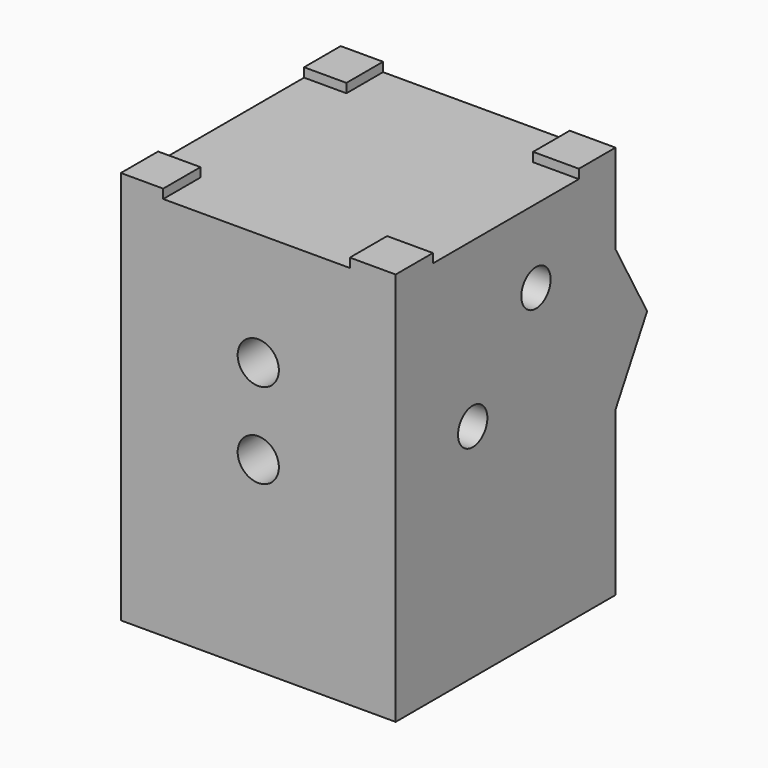
from build123d import *

# Parameters (mm, degrees)
F0_W      = 30
F0_H      = 30
F1_DEPTH  = 42
F5_R      = 2
F6_DEPTH  = 50
F8_R      = 2.25
F9_DEPTH  = 8
F10_R     = 2.25
F11_DEPTH = 16
F12_W     = 5
F12_H     = 5
F12_H_2   = 5.0838639587
F12_W_2   = 4.6232988685
F13_DEPTH = 1
F16_DEPTH = 20
F21_R     = 6.9
F2_R      = 6.75
F23_R     = 2.25
F24_DEPTH = 8.5855845434
F26_DEPTH = 30


with BuildPart() as f1:
    # F0 (on Top) → F1 (new body)
    with BuildSketch(Plane.XY):
        Rectangle(F0_W, F0_H)
    extrude(amount=F1_DEPTH)

    # F5 (on offset) → F6 (cut)
    with BuildSketch(Plane.YZ.offset(15)):
        with Locations((-4.4856271707, 24.1283942014)):
            Circle(F5_R)
        with Locations((4.1474616155, 33.9352041483)):
            Circle(F5_R)
    extrude(amount=-F6_DEPTH, mode=Mode.SUBTRACT)

    # F8 (on offset) → F9 (cut)
    with BuildSketch(Plane.XZ.offset(15)):
        with Locations((0, 20.3330869851)):
            Circle(F8_R)
    extrude(amount=-F9_DEPTH, mode=Mode.SUBTRACT)

    # F10 (on offset) → F11 (cut)
    with BuildSketch(Plane.XZ.offset(15)):
        with Locations((0, 29.6528354788)):
            Circle(F10_R)
    extrude(amount=-F11_DEPTH, mode=Mode.SUBTRACT)

    # F12 (on face) → F13 (join)
    with BuildSketch(Plane.XY.offset(42)):
        with Locations((12.5, 12.5)):
            Rectangle(F12_W, F12_H)
        with Locations((12.5, -12.4580680206)):
            Rectangle(F12_W, F12_H_2)
        with Locations((-12.6883505657, -12.4580680206)):
            Rectangle(F12_W_2, F12_H_2)
        with Locations((-12.6883505657, 12.5)):
            Rectangle(F12_W_2, F12_H)
    extrude(amount=F13_DEPTH)

    # F15 (on offset) → F16 (cut)
    with BuildSketch(Plane.YZ.offset(10)):
        with BuildLine():
            Line((-10.5428852386, 20.6804065085), (-6.3365916554, 16.9259020259))
            ThreePointArc((-6.3365916554, 16.9259020259), (0.0613537754, 26.1208148268), (8.0311429099, 33.9924466973))
            Line((8.0311429099, 33.9924466973), (4.3066875078, 37.316866219))
            Line((4.3066875078, 37.316866219), (-10.5428852386, 20.6804065085))
        make_face()
    extrude(amount=-F16_DEPTH, mode=Mode.SUBTRACT)

    # F17 (on Front) → F18 (revolve, cut)
    with BuildSketch(Plane.XZ):
        Polygon((10, 0), (0, 8.9987562969), (0, 0), align=None)
    revolve(axis=Axis((0, 0, 4.4993781485), (0, 0, 1)), mode=Mode.SUBTRACT)

    # F21 (on face) → F22 section 0
    with BuildSketch(Plane(origin=(0, -1.4039220881, 9.9894247186), x_dir=(1, 0, 0), z_dir=(0, -0.139173101, 0.9902680687))):
        with Locations((0, 1.4177192343)):
            Circle(F21_R)
    # F2 (on Top) → F22 section 1
    with BuildSketch(Plane.XY):
        Circle(F2_R)
    loft(mode=Mode.SUBTRACT)

    # F23 (on face) → F24 (cut, through all)
    with BuildSketch(Plane(origin=(0, 15, 0), x_dir=(-1, 0, 0), z_dir=(0, 1, 0))):
        with Locations((0, 6)):
            Circle(F23_R)
    extrude(amount=-F24_DEPTH, mode=Mode.SUBTRACT)

    # F25 (on face) → F26 (join)
    with BuildSketch(Plane.YZ.offset(15)):
        Polygon((19.3167924881, 25.5207791924), (15, 33.2272723317), (15, 17.8142860532), align=None)
    extrude(amount=-F26_DEPTH)


solid = f1.part
